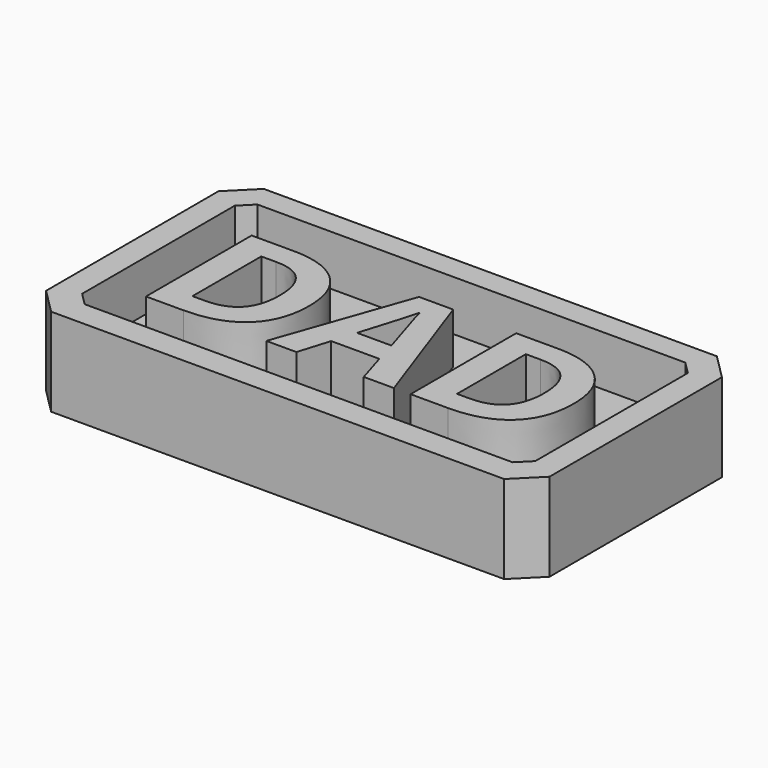
from build123d import *

# Parameters (mm, degrees)
F0_W         = 101.6
F0_H         = 53.6537654698
F1_DEPTH     = 7.62
F2_W         = 101.6
F2_H         = 53.6537654698
F2_W_2       = 91.44
F2_H_2       = 43.5792710632
F2_TEXT_SIZE = 37.3298887693
F3_DEPTH     = 10.16
F4_SIZE      = 5.08
F5_SIZE      = 2.54


# Not quite as in the source:
# - Text() gives the source's letters only with a copy of the font that has no kerning and outlines rounded to 1/6400 em; it was checked with that copy


with BuildPart() as f1:
    # F0 (on Top) → F1 (new body)
    with BuildSketch(Plane.XY):
        Rectangle(F0_W, F0_H)
    extrude(amount=F1_DEPTH)

    # F2 (on face) → F3 (join)
    with BuildSketch(Plane.XY.offset(7.62)):
        Rectangle(F2_W, F2_H)
        with Locations((0, 0.2494091168)):
            Rectangle(F2_W_2, F2_H_2, mode=Mode.SUBTRACT)
        with Locations((-40.64, -13.4387599569)):
            Text('DAD', F2_TEXT_SIZE, font='Open Sans', font_style=FontStyle.BOLD, text_align=(TextAlign.LEFT, TextAlign.BOTTOM))
    extrude(amount=F3_DEPTH)

    # F4
    f4_edges = [f1.edges().sort_by_distance(p)[0] for p in [
        (-50.8, -26.826883, 8.89),
        (-50.8, 26.826883, 8.89),
        (50.8, -26.826883, 8.89),
        (50.8, 26.826883, 8.89),
    ]]
    chamfer(f4_edges, length=F4_SIZE)

    # F5
    f5_edges = [f1.edges().sort_by_distance(p)[0] for p in [
        (45.72, 22.039045, 12.7),
        (45.72, -21.540226, 12.7),
        (-45.72, 22.039045, 12.7),
        (-45.72, -21.540226, 12.7),
    ]]
    chamfer(f5_edges, length=F5_SIZE)


solid = f1.part
